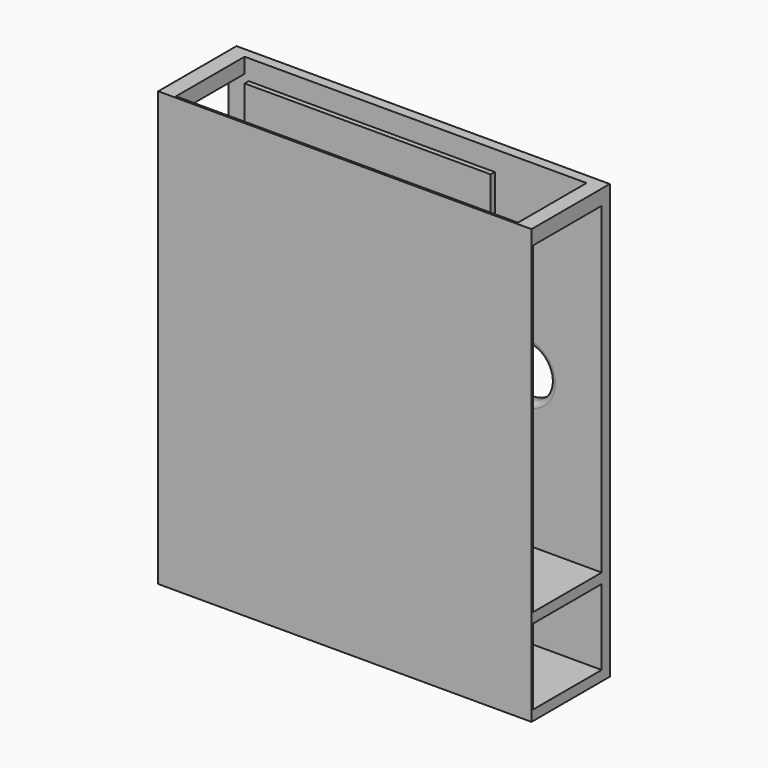
from build123d import *

# Parameters (mm, degrees)
F0_W      = 244
F0_H      = 305
F1_DEPTH  = 5
F2_W      = 370
F2_H      = 430
F4_DEPTH  = 10
F3_R      = 25
F5_DEPTH  = 12.5
F6_W      = 370
F6_H      = 10
F7_DEPTH  = 85
F8_W      = 370
F8_H      = 10
F9_DEPTH  = 85
F10_R     = 25
F11_DEPTH = 12.5
F13_R     = 4.99999
F12_W     = 15
F12_H     = 15
F12_W_2   = 16
F14_DEPTH = 85
F15_W     = 250
F15_H     = 30
F15_W_2   = 1.2186413854
F15_H_2   = 8.042093921
F16_DEPTH = 74
F17_W     = 120
F17_H     = 70
F18_DEPTH = 70
F19_W     = 370
F19_H     = 430
F20_DEPTH = 2


# Not quite as in the source:
# - a fillet or chamfer is up to 0.001 mm smaller than in the source, because OpenCascade refuses the exact size


with BuildPart() as f1:
    # F0 (on Front) → F1 (new body)
    with BuildSketch(Plane.XZ):
        with Locations((81.2744037509, 119.6701826155)):
            Rectangle(F0_W, F0_H)
        with BuildLine():
            Line((41.627296072, 179.8750311136), (39.4405335278, 179.8750311136))
            Line((39.4405335278, 179.8750311136), (31.5211831928, 200.5675271503))
            Line((31.5211831928, 200.5675271503), (31.3934517358, 200.5675271503))
            add(Edge.make_bspline(
                [(31.3934517358, 200.5675271503), (31.6182591002, 198.1099739173), (31.6182591002, 194.7225356772)],
                knots=[0, 0, 0, 1, 1, 1], degree=2))
            Line((31.6182591002, 194.7225356772), (31.6182591002, 179.8750311136))
            Line((31.6182591002, 179.8750311136), (29.1096132844, 179.8750311136))
            Line((29.1096132844, 179.8750311136), (29.1096132844, 203.2192321979))
            Line((29.1096132844, 203.2192321979), (33.1970199089, 203.2192321979))
            Line((33.1970199089, 203.2192321979), (40.590116641, 183.9624377381))
            Line((40.590116641, 183.9624377381), (40.717848098, 183.9624377381))
            Line((40.717848098, 183.9624377381), (48.1722559295, 203.2192321979))
            Line((48.1722559295, 203.2192321979), (52.2290070043, 203.2192321979))
            Line((52.2290070043, 203.2192321979), (52.2290070043, 179.8750311136))
            Line((52.2290070043, 179.8750311136), (49.5159908573, 179.8750311136))
            Line((49.5159908573, 179.8750311136), (49.5159908573, 194.9166874919))
            add(Edge.make_bspline(
                [(49.5159908573, 194.9166874919), (49.5159908573, 197.5019721819), (49.7407982216, 200.5368716006)],
                knots=[0, 0, 0, 1, 1, 1], degree=2))
            Line((49.7407982216, 200.5368716006), (49.6130667646, 200.5368716006))
            Line((49.6130667646, 200.5368716006), (41.627296072, 179.8750311136))
        make_face(mode=Mode.SUBTRACT)
        with BuildLine():
            add(Edge.make_bspline(
                [(71.1715820798, 195.2513439093), (73.3353529617, 192.806563822), (73.3353529617, 188.6425183232)],
                knots=[0, 0, 0, 1, 1, 1], degree=2))
            add(Edge.make_bspline(
                [(73.3353529617, 188.6425183232), (73.3353529617, 184.360959884), (71.1818005964, 181.957053863)],
                knots=[0, 0, 0, 1, 1, 1], degree=2))
            add(Edge.make_bspline(
                [(71.1818005964, 181.957053863), (69.0282482311, 179.5531478419), (65.2269600703, 179.5531478419)],
                knots=[0, 0, 0, 1, 1, 1], degree=2))
            add(Edge.make_bspline(
                [(65.2269600703, 179.5531478419), (62.8767012612, 179.5531478419), (61.0578053133, 180.6567476306)],
                knots=[0, 0, 0, 1, 1, 1], degree=2))
            add(Edge.make_bspline(
                [(61.0578053133, 180.6567476306), (59.2389093654, 181.7603474192), (58.2477132589, 183.8193785063)],
                knots=[0, 0, 0, 1, 1, 1], degree=2))
            add(Edge.make_bspline(
                [(58.2477132589, 183.8193785063), (57.2565171525, 185.8784095934), (57.2565171525, 188.6425183232)],
                knots=[0, 0, 0, 1, 1, 1], degree=2))
            add(Edge.make_bspline(
                [(57.2565171525, 188.6425183232), (57.2565171525, 192.9189675041), (59.3972963721, 195.3075457503)],
                knots=[0, 0, 0, 1, 1, 1], degree=2))
            add(Edge.make_bspline(
                [(59.3972963721, 195.3075457503), (61.5380755917, 197.6961239965), (65.3393637525, 197.6961239965)],
                knots=[0, 0, 0, 1, 1, 1], degree=2))
            add(Edge.make_bspline(
                [(65.3393637525, 197.6961239965), (69.007811198, 197.6961239965), (71.1715820798, 195.2513439093)],
                knots=[0, 0, 0, 1, 1, 1], degree=2))
        make_face(mode=Mode.SUBTRACT)
        with BuildLine():
            Line((90.2469978707, 179.8750311136), (89.8944590493, 182.2201806644))
            Line((89.8944590493, 182.2201806644), (89.7513998174, 182.2201806644))
            add(Edge.make_bspline(
                [(89.7513998174, 182.2201806644), (87.9171760947, 179.5531478419), (84.2589471657, 179.5531478419)],
                knots=[0, 0, 0, 1, 1, 1], degree=2))
            add(Edge.make_bspline(
                [(84.2589471657, 179.5531478419), (80.8255256011, 179.5531478419), (78.9172176333, 181.9008520219)],
                knots=[0, 0, 0, 1, 1, 1], degree=2))
            add(Edge.make_bspline(
                [(78.9172176333, 181.9008520219), (77.0089096655, 184.2485562019), (77.0089096655, 188.5760979656)],
                knots=[0, 0, 0, 1, 1, 1], degree=2))
            add(Edge.make_bspline(
                [(77.0089096655, 188.5760979656), (77.0089096655, 192.9036397293), (78.9248815207, 195.2998818629)],
                knots=[0, 0, 0, 1, 1, 1], degree=2))
            add(Edge.make_bspline(
                [(78.9248815207, 195.2998818629), (80.840853376, 197.6961239965), (84.2589471657, 197.6961239965)],
                knots=[0, 0, 0, 1, 1, 1], degree=2))
            add(Edge.make_bspline(
                [(84.2589471657, 197.6961239965), (87.8201001873, 197.6961239965), (89.7207442678, 195.1057300483)],
                knots=[0, 0, 0, 1, 1, 1], degree=2))
            Line((89.7207442678, 195.1057300483), (89.9302238573, 195.1057300483))
            Line((89.9302238573, 195.1057300483), (89.8178201751, 196.3677168436))
            Line((89.8178201751, 196.3677168436), (89.7513998174, 197.5990480892))
            Line((89.7513998174, 197.5990480892), (89.7513998174, 204.7213541324))
            Line((89.7513998174, 204.7213541324), (92.4031048651, 204.7213541324))
            Line((92.4031048651, 204.7213541324), (92.4031048651, 179.8750311136))
            Line((92.4031048651, 179.8750311136), (90.2469978707, 179.8750311136))
        make_face(mode=Mode.SUBTRACT)
        with BuildLine():
            add(Edge.make_bspline(
                [(108.4410666081, 179.8188292725), (107.1892983293, 179.5531478419), (105.4163857059, 179.5531478419)],
                knots=[0, 0, 0, 1, 1, 1], degree=2))
            add(Edge.make_bspline(
                [(105.4163857059, 179.5531478419), (101.5384586709, 179.5531478419), (99.2929396566, 181.9187344259)],
                knots=[0, 0, 0, 1, 1, 1], degree=2))
            add(Edge.make_bspline(
                [(99.2929396566, 181.9187344259), (97.0474206422, 184.2843210098), (97.0474206422, 188.4790220582)],
                knots=[0, 0, 0, 1, 1, 1], degree=2))
            add(Edge.make_bspline(
                [(97.0474206422, 188.4790220582), (97.0474206422, 192.7145971729), (99.1319980207, 195.2053605847)],
                knots=[0, 0, 0, 1, 1, 1], degree=2))
            add(Edge.make_bspline(
                [(99.1319980207, 195.2053605847), (101.2165753992, 197.6961239965), (104.7317450963, 197.6961239965)],
                knots=[0, 0, 0, 1, 1, 1], degree=2))
            add(Edge.make_bspline(
                [(104.7317450963, 197.6961239965), (108.0169981708, 197.6961239965), (109.932970026, 195.5323531147)],
                knots=[0, 0, 0, 1, 1, 1], degree=2))
            add(Edge.make_bspline(
                [(109.932970026, 195.5323531147), (111.8489418813, 193.3685822328), (111.8489418813, 189.8227569861)],
                knots=[0, 0, 0, 1, 1, 1], degree=2))
            Line((111.8489418813, 189.8227569861), (111.8489418813, 188.14692027))
            Line((111.8489418813, 188.14692027), (99.7962015972, 188.14692027))
            add(Edge.make_bspline(
                [(99.7962015972, 188.14692027), (99.8779497297, 185.0660375268), (101.3545253728, 183.4693943141)],
                knots=[0, 0, 0, 1, 1, 1], degree=2))
            add(Edge.make_bspline(
                [(101.3545253728, 183.4693943141), (102.8311010159, 181.8727511014), (105.5134616133, 181.8727511014)],
                knots=[0, 0, 0, 1, 1, 1], degree=2))
            add(Edge.make_bspline(
                [(105.5134616133, 181.8727511014), (108.3388814425, 181.8727511014), (111.097880914, 183.0529897642)],
                knots=[0, 0, 0, 1, 1, 1], degree=2))
            Line((111.097880914, 183.0529897642), (111.097880914, 180.6874031802))
            add(Edge.make_bspline(
                [(111.097880914, 180.6874031802), (109.6928348868, 180.0845107031), (108.4410666081, 179.8188292725)],
                knots=[0, 0, 0, 1, 1, 1], degree=2))
        make_face(mode=Mode.SUBTRACT)
        with BuildLine():
            Line((118.8639535006, 188.8315608796), (118.9916849576, 188.8315608796))
            add(Edge.make_bspline(
                [(118.9916849576, 188.8315608796), (119.6763255672, 189.8074292112), (121.0813715944, 191.3861900199)],
                knots=[0, 0, 0, 1, 1, 1], degree=2))
            Line((121.0813715944, 191.3861900199), (126.7322112528, 197.3742407249))
            Line((126.7322112528, 197.3742407249), (129.8795143537, 197.3742407249))
            Line((129.8795143537, 197.3742407249), (122.7878638601, 189.9198328934))
            Line((122.7878638601, 189.9198328934), (130.3751124069, 179.8750311136))
            Line((130.3751124069, 179.8750311136), (127.1664982067, 179.8750311136))
            Line((127.1664982067, 179.8750311136), (120.9842956871, 188.14692027))
            Line((120.9842956871, 188.14692027), (118.9916849576, 186.4199909711))
            Line((118.9916849576, 186.4199909711), (118.9916849576, 179.8750311136))
            Line((118.9916849576, 179.8750311136), (116.3706354596, 179.8750311136))
            Line((116.3706354596, 179.8750311136), (116.3706354596, 204.7213541324))
            Line((116.3706354596, 204.7213541324), (118.9916849576, 204.7213541324))
            Line((118.9916849576, 204.7213541324), (118.9916849576, 191.5445770266))
            add(Edge.make_bspline(
                [(118.9916849576, 191.5445770266), (118.9916849576, 190.6708938606), (118.8639535006, 188.8315608796)],
                knots=[0, 0, 0, 1, 1, 1], degree=2))
        make_face(mode=Mode.SUBTRACT)
        with BuildLine():
            add(Edge.make_bspline(
                [(146.4718306201, 195.2513439093), (148.635601502, 192.806563822), (148.635601502, 188.6425183232)],
                knots=[0, 0, 0, 1, 1, 1], degree=2))
            add(Edge.make_bspline(
                [(148.635601502, 188.6425183232), (148.635601502, 184.360959884), (146.4820491367, 181.957053863)],
                knots=[0, 0, 0, 1, 1, 1], degree=2))
            add(Edge.make_bspline(
                [(146.4820491367, 181.957053863), (144.3284967714, 179.5531478419), (140.5272086106, 179.5531478419)],
                knots=[0, 0, 0, 1, 1, 1], degree=2))
            add(Edge.make_bspline(
                [(140.5272086106, 179.5531478419), (138.1769498015, 179.5531478419), (136.3580538536, 180.6567476306)],
                knots=[0, 0, 0, 1, 1, 1], degree=2))
            add(Edge.make_bspline(
                [(136.3580538536, 180.6567476306), (134.5391579056, 181.7603474192), (133.5479617992, 183.8193785063)],
                knots=[0, 0, 0, 1, 1, 1], degree=2))
            add(Edge.make_bspline(
                [(133.5479617992, 183.8193785063), (132.5567656927, 185.8784095934), (132.5567656927, 188.6425183232)],
                knots=[0, 0, 0, 1, 1, 1], degree=2))
            add(Edge.make_bspline(
                [(132.5567656927, 188.6425183232), (132.5567656927, 192.9189675041), (134.6975449123, 195.3075457503)],
                knots=[0, 0, 0, 1, 1, 1], degree=2))
            add(Edge.make_bspline(
                [(134.6975449123, 195.3075457503), (136.8383241319, 197.6961239965), (140.6396122927, 197.6961239965)],
                knots=[0, 0, 0, 1, 1, 1], degree=2))
            add(Edge.make_bspline(
                [(140.6396122927, 197.6961239965), (144.3080597383, 197.6961239965), (146.4718306201, 195.2513439093)],
                knots=[0, 0, 0, 1, 1, 1], degree=2))
        make_face(mode=Mode.SUBTRACT)
        with BuildLine():
            add(Edge.make_bspline(
                [(158.2512255862, 196.7687936186), (159.6256160636, 197.6961239965), (161.27079723, 197.6961239965)],
                knots=[0, 0, 0, 1, 1, 1], degree=2))
            add(Edge.make_bspline(
                [(161.27079723, 197.6961239965), (162.435708118, 197.6961239965), (163.3604838668, 197.5019721819)],
                knots=[0, 0, 0, 1, 1, 1], degree=2))
            Line((163.3604838668, 197.5019721819), (162.9926172706, 195.0444189489))
            add(Edge.make_bspline(
                [(162.9926172706, 195.0444189489), (161.9094545151, 195.2845540881), (161.0766454154, 195.2845540881)],
                knots=[0, 0, 0, 1, 1, 1], degree=2))
            add(Edge.make_bspline(
                [(161.0766454154, 195.2845540881), (158.9511939706, 195.2845540881), (157.4439627778, 193.5601794184)],
                knots=[0, 0, 0, 1, 1, 1], degree=2))
            add(Edge.make_bspline(
                [(157.4439627778, 193.5601794184), (155.936731585, 191.8358047486), (155.936731585, 189.2658478335)],
                knots=[0, 0, 0, 1, 1, 1], degree=2))
            Line((155.936731585, 189.2658478335), (155.936731585, 179.8750311136))
            Line((155.936731585, 179.8750311136), (153.2850265374, 179.8750311136))
            Line((153.2850265374, 179.8750311136), (153.2850265374, 197.3742407249))
            Line((153.2850265374, 197.3742407249), (155.4717890815, 197.3742407249))
            Line((155.4717890815, 197.3742407249), (155.7783445783, 194.1349709749))
            Line((155.7783445783, 194.1349709749), (155.9060760353, 194.1349709749))
            add(Edge.make_bspline(
                [(155.9060760353, 194.1349709749), (156.8768351087, 195.8414632407), (158.2512255862, 196.7687936186)],
                knots=[0, 0, 0, 1, 1, 1], degree=2))
        make_face(mode=Mode.SUBTRACT)
        with BuildLine():
            add(Edge.make_bspline(
                [(170.227326996, 182.5906018898), (170.9783879633, 181.7450196443), (172.2863580831, 181.7450196443)],
                knots=[0, 0, 0, 1, 1, 1], degree=2))
            add(Edge.make_bspline(
                [(172.2863580831, 181.7450196443), (172.9914357258, 181.7450196443), (173.6454207858, 181.84720481)],
                knots=[0, 0, 0, 1, 1, 1], degree=2))
            add(Edge.make_bspline(
                [(173.6454207858, 181.84720481), (174.2994058457, 181.9493899756), (174.6826002167, 182.0617936577)],
                knots=[0, 0, 0, 1, 1, 1], degree=2))
            Line((174.6826002167, 182.0617936577), (174.6826002167, 180.0334181203))
            add(Edge.make_bspline(
                [(174.6826002167, 180.0334181203), (174.2534225212, 179.8290477891), (173.4155041631, 179.6910978155)],
                knots=[0, 0, 0, 1, 1, 1], degree=2))
            add(Edge.make_bspline(
                [(173.4155041631, 179.6910978155), (172.5775858051, 179.5531478419), (171.9031637121, 179.5531478419)],
                knots=[0, 0, 0, 1, 1, 1], degree=2))
            add(Edge.make_bspline(
                [(171.9031637121, 179.5531478419), (166.8296702394, 179.5531478419), (166.8296702394, 184.9025412618)],
                knots=[0, 0, 0, 1, 1, 1], degree=2))
            Line((166.8296702394, 184.9025412618), (166.8296702394, 195.3152096378))
            Line((166.8296702394, 195.3152096378), (164.3210244236, 195.3152096378))
            Line((164.3210244236, 195.3152096378), (164.3210244236, 196.5925242079))
            Line((164.3210244236, 196.5925242079), (166.8296702394, 197.6961239965))
            Line((166.8296702394, 197.6961239965), (167.9434885446, 201.4309917997))
            Line((167.9434885446, 201.4309917997), (169.4762660287, 201.4309917997))
            Line((169.4762660287, 201.4309917997), (169.4762660287, 197.3742407249))
            Line((169.4762660287, 197.3742407249), (174.5548687597, 197.3742407249))
            Line((174.5548687597, 197.3742407249), (174.5548687597, 195.3152096378))
            Line((174.5548687597, 195.3152096378), (169.4762660287, 195.3152096378))
            Line((169.4762660287, 195.3152096378), (169.4762660287, 185.014944944))
            add(Edge.make_bspline(
                [(169.4762660287, 185.014944944), (169.4762660287, 183.4361841352), (170.227326996, 182.5906018898)],
                knots=[0, 0, 0, 1, 1, 1], degree=2))
        make_face(mode=Mode.SUBTRACT)
    extrude(amount=F1_DEPTH)

    # F2 (on Front) → F4 (join)
    with BuildSketch(Plane.XZ):
        with Locations((124.2744037509, 77.1701826155)):
            Rectangle(F2_W, F2_H)
    extrude(amount=-F4_DEPTH)

    # F3 (on Front) → F5 (cut, symmetric)
    with BuildSketch(Plane.XZ):
        with Locations((233.2744037509, 107.1701826155)):
            Circle(F3_R)
    extrude(amount=F5_DEPTH, both=True, mode=Mode.SUBTRACT)

    # F6 (on Front) → F7 (join)
    with BuildSketch(Plane.XZ):
        with Locations((124.2744037509, -47.8298173845)):
            Rectangle(F6_W, F6_H)
    extrude(amount=F7_DEPTH)

    # F8 (on Front) → F9 (join)
    with BuildSketch(Plane.XZ):
        with Locations((124.2744037509, -132.8298173845)):
            Rectangle(F8_W, F8_H)
    extrude(amount=F9_DEPTH)

    # F10 (on Front) → F11 (cut, symmetric)
    with BuildSketch(Plane.XZ):
        with Locations((149.9174684286, -85.3298173845)):
            Circle(F10_R)
    extrude(amount=F11_DEPTH, both=True, mode=Mode.SUBTRACT)

    # F13 (radius 5 in the source; OpenCascade refuses exactly that, so slightly less here)
    f13_edges = [f1.edges().sort_by_distance(p)[0] for p in [
        (208.274404, 0, 107.170183),
        (124.917468, 0, -85.329817),
    ]]
    fillet(f13_edges, radius=F13_R)

    # F12 (on Front) → F14 (join)
    with BuildSketch(Plane.XZ):
        with Locations((301.7744037509, 284.6701826155)):
            Rectangle(F12_W, F12_H)
        with Locations((-52.7255962491, 284.6701826155)):
            Rectangle(F12_W_2, F12_H)
    extrude(amount=F14_DEPTH)

    # F15 (on face) → F16 (join)
    with BuildSketch(Plane.XZ.offset(5)):
        with Locations((84.2744037509, 79.079321873)):
            Rectangle(F15_W, F15_H)
        with BuildLine():
            add(Edge.make_bspline(
                [(24.3571698455, 81.6391274461), (24.9887970761, 82.0652997225), (25.7448713075, 82.0652997225)],
                knots=[0, 0, 0, 1, 1, 1], degree=2))
            add(Edge.make_bspline(
                [(25.7448713075, 82.0652997225), (26.2802282167, 82.0652997225), (26.7052264648, 81.9760735709)],
                knots=[0, 0, 0, 1, 1, 1], degree=2))
            Line((26.7052264648, 81.9760735709), (26.5361663882, 80.8466583371))
            add(Edge.make_bspline(
                [(26.5361663882, 80.8466583371), (26.0383783849, 80.9570169982), (25.655645156, 80.9570169982)],
                knots=[0, 0, 0, 1, 1, 1], degree=2))
            add(Edge.make_bspline(
                [(25.655645156, 80.9570169982), (24.6788536024, 80.9570169982), (23.9861768997, 80.1645478892)],
                knots=[0, 0, 0, 1, 1, 1], degree=2))
            add(Edge.make_bspline(
                [(23.9861768997, 80.1645478892), (23.293500197, 79.3720787802), (23.293500197, 78.1910063007)],
                knots=[0, 0, 0, 1, 1, 1], degree=2))
            Line((23.293500197, 78.1910063007), (23.293500197, 73.8752782345))
            Line((23.293500197, 73.8752782345), (22.0748588116, 73.8752782345))
            Line((22.0748588116, 73.8752782345), (22.0748588116, 81.9173721555))
            Line((22.0748588116, 81.9173721555), (23.0798270447, 81.9173721555))
            Line((23.0798270447, 81.9173721555), (23.2207104418, 80.4287042588))
            Line((23.2207104418, 80.4287042588), (23.2794118573, 80.4287042588))
            add(Edge.make_bspline(
                [(23.2794118573, 80.4287042588), (23.725542615, 81.2129551697), (24.3571698455, 81.6391274461)],
                knots=[0, 0, 0, 1, 1, 1], degree=2))
        make_face(mode=Mode.SUBTRACT)
        with BuildLine():
            Line((34.0593397963, 73.8752782345), (33.1553379979, 73.8752782345))
            Line((33.1553379979, 73.8752782345), (32.9134881661, 75.0211298647))
            Line((32.9134881661, 75.0211298647), (32.8547867507, 75.0211298647))
            add(Edge.make_bspline(
                [(32.8547867507, 75.0211298647), (32.2536842561, 74.2650556333), (31.6561038465, 73.9962031504)],
                knots=[0, 0, 0, 1, 1, 1], degree=2))
            add(Edge.make_bspline(
                [(31.6561038465, 73.9962031504), (31.0585234369, 73.7273506675), (30.1615658084, 73.7273506675)],
                knots=[0, 0, 0, 1, 1, 1], degree=2))
            add(Edge.make_bspline(
                [(30.1615658084, 73.7273506675), (28.9664049892, 73.7273506675), (28.2878166262, 74.3448895583)],
                knots=[0, 0, 0, 1, 1, 1], degree=2))
            add(Edge.make_bspline(
                [(28.2878166262, 74.3448895583), (27.6092282632, 74.9624284492), (27.6092282632, 76.0988878529)],
                knots=[0, 0, 0, 1, 1, 1], degree=2))
            add(Edge.make_bspline(
                [(27.6092282632, 76.0988878529), (27.6092282632, 78.5338225671), (31.5046541946, 78.6512253981)],
                knots=[0, 0, 0, 1, 1, 1], degree=2))
            Line((31.5046541946, 78.6512253981), (32.8688750904, 78.6958384738))
            Line((32.8688750904, 78.6958384738), (32.8688750904, 79.1959745337))
            add(Edge.make_bspline(
                [(32.8688750904, 79.1959745337), (32.8688750904, 80.1422413513), (32.4626612952, 80.5930682222)],
                knots=[0, 0, 0, 1, 1, 1], degree=2))
            add(Edge.make_bspline(
                [(32.4626612952, 80.5930682222), (32.0564475001, 81.0438950931), (31.1594898715, 81.0438950931)],
                knots=[0, 0, 0, 1, 1, 1], degree=2))
            add(Edge.make_bspline(
                [(31.1594898715, 81.0438950931), (30.1545216385, 81.0438950931), (28.8865710641, 80.4287042588)],
                knots=[0, 0, 0, 1, 1, 1], degree=2))
            Line((28.8865710641, 80.4287042588), (28.510882005, 81.3608827367))
            add(Edge.make_bspline(
                [(28.510882005, 81.3608827367), (29.1049403297, 81.6825664935), (29.8128794004, 81.8657149098)],
                knots=[0, 0, 0, 1, 1, 1], degree=2))
            add(Edge.make_bspline(
                [(29.8128794004, 81.8657149098), (30.5208184711, 82.0488633261), (31.2346276834, 82.0488633261)],
                knots=[0, 0, 0, 1, 1, 1], degree=2))
            add(Edge.make_bspline(
                [(31.2346276834, 82.0488633261), (32.6716383344, 82.0488633261), (33.3654890653, 81.411365954)],
                knots=[0, 0, 0, 1, 1, 1], degree=2))
            add(Edge.make_bspline(
                [(33.3654890653, 81.411365954), (34.0593397963, 80.7738685819), (34.0593397963, 79.3650346103)],
                knots=[0, 0, 0, 1, 1, 1], degree=2))
            Line((34.0593397963, 79.3650346103), (34.0593397963, 73.8752782345))
        make_face(mode=Mode.SUBTRACT)
        with Locations((42.2693197656, 77.896325195)):
            Rectangle(F15_W_2, F15_H_2, mode=Mode.SUBTRACT)
        with BuildLine():
            add(Edge.make_bspline(
                [(67.182200496, 80.9417546302), (68.1766024742, 79.8182095378), (68.1766024742, 77.9045433931)],
                knots=[0, 0, 0, 1, 1, 1], degree=2))
            add(Edge.make_bspline(
                [(68.1766024742, 77.9045433931), (68.1766024742, 75.9368719462), (67.1868966092, 74.8321113068)],
                knots=[0, 0, 0, 1, 1, 1], degree=2))
            add(Edge.make_bspline(
                [(67.1868966092, 74.8321113068), (66.1971907442, 73.7273506675), (64.4502366195, 73.7273506675)],
                knots=[0, 0, 0, 1, 1, 1], degree=2))
            add(Edge.make_bspline(
                [(64.4502366195, 73.7273506675), (63.3701305746, 73.7273506675), (62.5342224181, 74.2345308972)],
                knots=[0, 0, 0, 1, 1, 1], degree=2))
            add(Edge.make_bspline(
                [(62.5342224181, 74.2345308972), (61.6983142617, 74.741711127), (61.2427912775, 75.6879779446)],
                knots=[0, 0, 0, 1, 1, 1], degree=2))
            add(Edge.make_bspline(
                [(61.2427912775, 75.6879779446), (60.7872682934, 76.6342447621), (60.7872682934, 77.9045433931)],
                knots=[0, 0, 0, 1, 1, 1], degree=2))
            add(Edge.make_bspline(
                [(60.7872682934, 77.9045433931), (60.7872682934, 79.8698667835), (61.7711040169, 80.967583253)],
                knots=[0, 0, 0, 1, 1, 1], degree=2))
            add(Edge.make_bspline(
                [(61.7711040169, 80.967583253), (62.7549397403, 82.0652997225), (64.5018938651, 82.0652997225)],
                knots=[0, 0, 0, 1, 1, 1], degree=2))
            add(Edge.make_bspline(
                [(64.5018938651, 82.0652997225), (66.1877985177, 82.0652997225), (67.182200496, 80.9417546302)],
                knots=[0, 0, 0, 1, 1, 1], degree=2))
        make_face(mode=Mode.SUBTRACT)
        with BuildLine():
            add(Edge.make_bspline(
                [(72.5956450317, 81.6391274461), (73.2272722623, 82.0652997225), (73.9833464937, 82.0652997225)],
                knots=[0, 0, 0, 1, 1, 1], degree=2))
            add(Edge.make_bspline(
                [(73.9833464937, 82.0652997225), (74.5187034028, 82.0652997225), (74.9437016509, 81.9760735709)],
                knots=[0, 0, 0, 1, 1, 1], degree=2))
            Line((74.9437016509, 81.9760735709), (74.7746415743, 80.8466583371))
            add(Edge.make_bspline(
                [(74.7746415743, 80.8466583371), (74.2768535711, 80.9570169982), (73.8941203421, 80.9570169982)],
                knots=[0, 0, 0, 1, 1, 1], degree=2))
            add(Edge.make_bspline(
                [(73.8941203421, 80.9570169982), (72.9173287885, 80.9570169982), (72.2246520858, 80.1645478892)],
                knots=[0, 0, 0, 1, 1, 1], degree=2))
            add(Edge.make_bspline(
                [(72.2246520858, 80.1645478892), (71.5319753831, 79.3720787802), (71.5319753831, 78.1910063007)],
                knots=[0, 0, 0, 1, 1, 1], degree=2))
            Line((71.5319753831, 78.1910063007), (71.5319753831, 73.8752782345))
            Line((71.5319753831, 73.8752782345), (70.3133339977, 73.8752782345))
            Line((70.3133339977, 73.8752782345), (70.3133339977, 81.9173721555))
            Line((70.3133339977, 81.9173721555), (71.3183022308, 81.9173721555))
            Line((71.3183022308, 81.9173721555), (71.4591856279, 80.4287042588))
            Line((71.4591856279, 80.4287042588), (71.5178870434, 80.4287042588))
            add(Edge.make_bspline(
                [(71.5178870434, 80.4287042588), (71.9640178011, 81.2129551697), (72.5956450317, 81.6391274461)],
                knots=[0, 0, 0, 1, 1, 1], degree=2))
        make_face(mode=Mode.SUBTRACT)
        with BuildLine():
            add(Edge.make_bspline(
                [(78.0994897472, 75.1232703276), (78.4446540703, 74.7346669571), (79.0457565648, 74.7346669571)],
                knots=[0, 0, 0, 1, 1, 1], degree=2))
            add(Edge.make_bspline(
                [(79.0457565648, 74.7346669571), (79.3697883782, 74.7346669571), (79.6703396255, 74.7816280895)],
                knots=[0, 0, 0, 1, 1, 1], degree=2))
            add(Edge.make_bspline(
                [(79.6703396255, 74.7816280895), (79.9708908728, 74.8285892219), (80.1469951192, 74.8802464675)],
                knots=[0, 0, 0, 1, 1, 1], degree=2))
            Line((80.1469951192, 74.8802464675), (80.1469951192, 73.9480679897))
            add(Edge.make_bspline(
                [(80.1469951192, 73.9480679897), (79.9497583632, 73.8541457249), (79.5646770776, 73.7907481962)],
                knots=[0, 0, 0, 1, 1, 1], degree=2))
            add(Edge.make_bspline(
                [(79.5646770776, 73.7907481962), (79.1795957921, 73.7273506675), (78.8696523183, 73.7273506675)],
                knots=[0, 0, 0, 1, 1, 1], degree=2))
            add(Edge.make_bspline(
                [(78.8696523183, 73.7273506675), (76.5380320954, 73.7273506675), (76.5380320954, 76.1857659478)],
                knots=[0, 0, 0, 1, 1, 1], degree=2))
            Line((76.5380320954, 76.1857659478), (76.5380320954, 80.9711053379))
            Line((76.5380320954, 80.9711053379), (75.3851362954, 80.9711053379))
            Line((75.3851362954, 80.9711053379), (75.3851362954, 81.5581194927))
            Line((75.3851362954, 81.5581194927), (76.5380320954, 82.0652997225))
            Line((76.5380320954, 82.0652997225), (77.0499084384, 83.7817291112))
            Line((77.0499084384, 83.7817291112), (77.7543254242, 83.7817291112))
            Line((77.7543254242, 83.7817291112), (77.7543254242, 81.9173721555))
            Line((77.7543254242, 81.9173721555), (80.0882937037, 81.9173721555))
            Line((80.0882937037, 81.9173721555), (80.0882937037, 80.9711053379))
            Line((80.0882937037, 80.9711053379), (77.7543254242, 80.9711053379))
            Line((77.7543254242, 80.9711053379), (77.7543254242, 76.2374231935))
            add(Edge.make_bspline(
                [(77.7543254242, 76.2374231935), (77.7543254242, 75.5118736981), (78.0994897472, 75.1232703276)],
                knots=[0, 0, 0, 1, 1, 1], degree=2))
        make_face(mode=Mode.SUBTRACT)
        with BuildLine():
            Line((16.0380052435, 78.3811988868), (16.0380052435, 79.496525781))
            Line((16.0380052435, 79.496525781), (19.6845371732, 79.496525781))
            Line((19.6845371732, 79.496525781), (19.6845371732, 74.279143973))
            add(Edge.make_bspline(
                [(19.6845371732, 74.279143973), (18.8321926204, 74.0067694052), (17.9516713882, 73.8670600363)],
                knots=[0, 0, 0, 1, 1, 1], degree=2))
            add(Edge.make_bspline(
                [(17.9516713882, 73.8670600363), (17.071150156, 73.7273506675), (15.9112101861, 73.7273506675)],
                knots=[0, 0, 0, 1, 1, 1], degree=2))
            add(Edge.make_bspline(
                [(15.9112101861, 73.7273506675), (13.4762754719, 73.7273506675), (12.1190987459, 75.1772756299)],
                knots=[0, 0, 0, 1, 1, 1], degree=2))
            add(Edge.make_bspline(
                [(12.1190987459, 75.1772756299), (10.76192202, 76.6272005923), (10.76192202, 79.2382395529)],
                knots=[0, 0, 0, 1, 1, 1], degree=2))
            add(Edge.make_bspline(
                [(10.76192202, 79.2382395529), (10.76192202, 80.9124039224), (11.4334662131, 82.1709622703)],
                knots=[0, 0, 0, 1, 1, 1], degree=2))
            add(Edge.make_bspline(
                [(11.4334662131, 82.1709622703), (12.1050104062, 83.4295206183), (13.3670908391, 84.0928466132)],
                knots=[0, 0, 0, 1, 1, 1], degree=2))
            add(Edge.make_bspline(
                [(13.3670908391, 84.0928466132), (14.6291712719, 84.7561726081), (16.3221200944, 84.7561726081)],
                knots=[0, 0, 0, 1, 1, 1], degree=2))
            add(Edge.make_bspline(
                [(16.3221200944, 84.7561726081), (18.0408975397, 84.7561726081), (19.5225212665, 84.1268934342)],
                knots=[0, 0, 0, 1, 1, 1], degree=2))
            Line((19.5225212665, 84.1268934342), (19.0388216029, 83.0256548797))
            add(Edge.make_bspline(
                [(19.0388216029, 83.0256548797), (17.5853745556, 83.640845714), (16.2422861694, 83.640845714)],
                knots=[0, 0, 0, 1, 1, 1], degree=2))
            add(Edge.make_bspline(
                [(16.2422861694, 83.640845714), (14.2840069489, 83.640845714), (13.1827683945, 82.4750356025)],
                knots=[0, 0, 0, 1, 1, 1], degree=2))
            add(Edge.make_bspline(
                [(13.1827683945, 82.4750356025), (12.08152984, 81.3092254911), (12.08152984, 79.2382395529)],
                knots=[0, 0, 0, 1, 1, 1], degree=2))
            add(Edge.make_bspline(
                [(12.08152984, 79.2382395529), (12.08152984, 77.0662871801), (13.1416774036, 75.9439161161)],
                knots=[0, 0, 0, 1, 1, 1], degree=2))
            add(Edge.make_bspline(
                [(13.1416774036, 75.9439161161), (14.2018249672, 74.821545052), (16.2563745091, 74.821545052)],
                knots=[0, 0, 0, 1, 1, 1], degree=2))
            add(Edge.make_bspline(
                [(16.2563745091, 74.821545052), (17.3717014032, 74.821545052), (18.4353710518, 75.0798312802)],
                knots=[0, 0, 0, 1, 1, 1], degree=2))
            Line((18.4353710518, 75.0798312802), (18.4353710518, 78.3811988868))
            Line((18.4353710518, 78.3811988868), (16.0380052435, 78.3811988868))
        make_face(mode=Mode.SUBTRACT)
        with BuildLine():
            Line((40.1924636858, 81.9173721555), (40.1924636858, 80.9711053379))
            Line((40.1924636858, 80.9711053379), (38.1449583139, 80.9711053379))
            Line((38.1449583139, 80.9711053379), (38.1449583139, 73.8752782345))
            Line((38.1449583139, 73.8752782345), (36.9263169285, 73.8752782345))
            Line((36.9263169285, 73.8752782345), (36.9263169285, 80.9711053379))
            Line((36.9263169285, 80.9711053379), (35.4893062775, 80.9711053379))
            Line((35.4893062775, 80.9711053379), (35.4893062775, 81.5205505868))
            Line((35.4893062775, 81.5205505868), (36.9263169285, 81.9619852312))
            Line((36.9263169285, 81.9619852312), (36.9263169285, 82.4081159889))
            add(Edge.make_bspline(
                [(36.9263169285, 82.4081159889), (36.9263169285, 85.373711499), (39.5162233795, 85.373711499)],
                knots=[0, 0, 0, 1, 1, 1], degree=2))
            add(Edge.make_bspline(
                [(39.5162233795, 85.373711499), (40.1548947799, 85.373711499), (41.0142835026, 85.1177733275)],
                knots=[0, 0, 0, 1, 1, 1], degree=2))
            Line((41.0142835026, 85.1177733275), (40.697295859, 84.1409817739))
            add(Edge.make_bspline(
                [(40.697295859, 84.1409817739), (39.9928788732, 84.368743266), (39.4950908699, 84.368743266)],
                knots=[0, 0, 0, 1, 1, 1], degree=2))
            add(Edge.make_bspline(
                [(39.4950908699, 84.368743266), (38.8047622239, 84.368743266), (38.4748602689, 83.9096981969)],
                knots=[0, 0, 0, 1, 1, 1], degree=2))
            add(Edge.make_bspline(
                [(38.4748602689, 83.9096981969), (38.1449583139, 83.4506531278), (38.1449583139, 82.4386407249)],
                knots=[0, 0, 0, 1, 1, 1], degree=2))
            Line((38.1449583139, 82.4386407249), (38.1449583139, 81.9173721555))
            Line((38.1449583139, 81.9173721555), (40.1924636858, 81.9173721555))
        make_face(mode=Mode.SUBTRACT)
        with BuildLine():
            Line((46.6073543697, 77.991421488), (46.6660557852, 77.991421488))
            add(Edge.make_bspline(
                [(46.6660557852, 77.991421488), (46.9806953721, 78.4399003023), (47.6264109424, 79.1654497977)],
                knots=[0, 0, 0, 1, 1, 1], degree=2))
            Line((47.6264109424, 79.1654497977), (50.2233615633, 81.9173721555))
            Line((50.2233615633, 81.9173721555), (51.6697644408, 81.9173721555))
            Line((51.6697644408, 81.9173721555), (48.4106618533, 78.491557548))
            Line((48.4106618533, 78.491557548), (51.8975259329, 73.8752782345))
            Line((51.8975259329, 73.8752782345), (50.422946376, 73.8752782345))
            Line((50.422946376, 73.8752782345), (47.5817978667, 77.6767819011))
            Line((47.5817978667, 77.6767819011), (46.6660557852, 76.8831387638))
            Line((46.6660557852, 76.8831387638), (46.6660557852, 73.8752782345))
            Line((46.6660557852, 73.8752782345), (45.4615027395, 73.8752782345))
            Line((45.4615027395, 73.8752782345), (45.4615027395, 85.293877574))
            Line((45.4615027395, 85.293877574), (46.6660557852, 85.293877574))
            Line((46.6660557852, 85.293877574), (46.6660557852, 79.2382395529))
            add(Edge.make_bspline(
                [(46.6660557852, 79.2382395529), (46.6660557852, 78.836721871), (46.6073543697, 77.991421488)],
                knots=[0, 0, 0, 1, 1, 1], degree=2))
        make_face(mode=Mode.SUBTRACT)
        with BuildLine():
            Line((54.4944765538, 77.991421488), (54.5531779693, 77.991421488))
            add(Edge.make_bspline(
                [(54.5531779693, 77.991421488), (54.8678175562, 78.4399003023), (55.5135331265, 79.1654497977)],
                knots=[0, 0, 0, 1, 1, 1], degree=2))
            Line((55.5135331265, 79.1654497977), (58.1104837474, 81.9173721555))
            Line((58.1104837474, 81.9173721555), (59.5568866249, 81.9173721555))
            Line((59.5568866249, 81.9173721555), (56.2977840374, 78.491557548))
            Line((56.2977840374, 78.491557548), (59.784648117, 73.8752782345))
            Line((59.784648117, 73.8752782345), (58.3100685601, 73.8752782345))
            Line((58.3100685601, 73.8752782345), (55.4689200508, 77.6767819011))
            Line((55.4689200508, 77.6767819011), (54.5531779693, 76.8831387638))
            Line((54.5531779693, 76.8831387638), (54.5531779693, 73.8752782345))
            Line((54.5531779693, 73.8752782345), (53.3486249236, 73.8752782345))
            Line((53.3486249236, 73.8752782345), (53.3486249236, 85.293877574))
            Line((53.3486249236, 85.293877574), (54.5531779693, 85.293877574))
            Line((54.5531779693, 85.293877574), (54.5531779693, 79.2382395529))
            add(Edge.make_bspline(
                [(54.5531779693, 79.2382395529), (54.5531779693, 78.836721871), (54.4944765538, 77.991421488)],
                knots=[0, 0, 0, 1, 1, 1], degree=2))
        make_face(mode=Mode.SUBTRACT)
        with BuildLine():
            add(Edge.make_bspline(
                [(41.7621395358, 83.4835259205), (41.5566845816, 83.6854587898), (41.5566845816, 84.0963686981)],
                knots=[0, 0, 0, 1, 1, 1], degree=2))
            add(Edge.make_bspline(
                [(41.5566845816, 84.0963686981), (41.5566845816, 84.5143227764), (41.7621395358, 84.7092114758)],
                knots=[0, 0, 0, 1, 1, 1], degree=2))
            add(Edge.make_bspline(
                [(41.7621395358, 84.7092114758), (41.96759449, 84.9041001752), (42.2775379638, 84.9041001752)],
                knots=[0, 0, 0, 1, 1, 1], degree=2))
            add(Edge.make_bspline(
                [(42.2775379638, 84.9041001752), (42.5710450412, 84.9041001752), (42.7835441652, 84.7056893908)],
                knots=[0, 0, 0, 1, 1, 1], degree=2))
            add(Edge.make_bspline(
                [(42.7835441652, 84.7056893908), (42.9960432892, 84.5072786065), (42.9960432892, 84.0963686981)],
                knots=[0, 0, 0, 1, 1, 1], degree=2))
            add(Edge.make_bspline(
                [(42.9960432892, 84.0963686981), (42.9960432892, 83.6854587898), (42.7835441652, 83.4835259205)],
                knots=[0, 0, 0, 1, 1, 1], degree=2))
            add(Edge.make_bspline(
                [(42.7835441652, 83.4835259205), (42.5710450412, 83.2815930512), (42.2775379638, 83.2815930512)],
                knots=[0, 0, 0, 1, 1, 1], degree=2))
            add(Edge.make_bspline(
                [(42.2775379638, 83.2815930512), (41.96759449, 83.2815930512), (41.7621395358, 83.4835259205)],
                knots=[0, 0, 0, 1, 1, 1], degree=2))
        make_face(mode=Mode.SUBTRACT)
    extrude(amount=F16_DEPTH)

    # F17 (on Front) → F18 (join)
    with BuildSketch(Plane.XZ):
        with Locations((-0.7255962491, -92.8298173845)):
            Rectangle(F17_W, F17_H)
    extrude(amount=F18_DEPTH)

    # F19 (on face) → F20 (join)
    with BuildSketch(Plane.XZ.offset(85)):
        with Locations((124.2744037509, 77.1701826155)):
            Rectangle(F19_W, F19_H)
    extrude(amount=F20_DEPTH)


solid = f1.part
